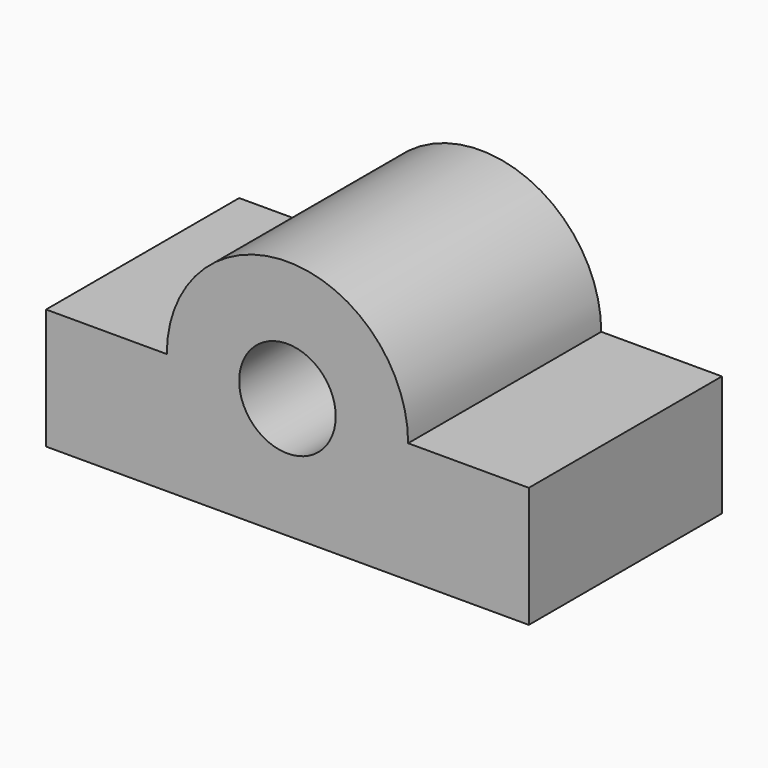
from build123d import *

# Parameters (mm, degrees)
F0_R     = 304.8
F1_DEPTH = 762


with BuildPart() as f1:
    # F0 (on Front) → F1 (new body, symmetric)
    with BuildSketch(Plane.XZ):
        with BuildLine():
            Line((1524, 0), (762, 0))
            ThreePointArc((762, 0), (0, 762), (-762, 0))
            Line((-762, 0), (-1524, 0))
            Line((-1524, 0), (-1524, -762))
            Line((-1524, -762), (1524, -762))
            Line((1524, -762), (1524, 0))
        make_face()
        Circle(F0_R, mode=Mode.SUBTRACT)
    extrude(amount=F1_DEPTH, both=True)


solid = f1.part
